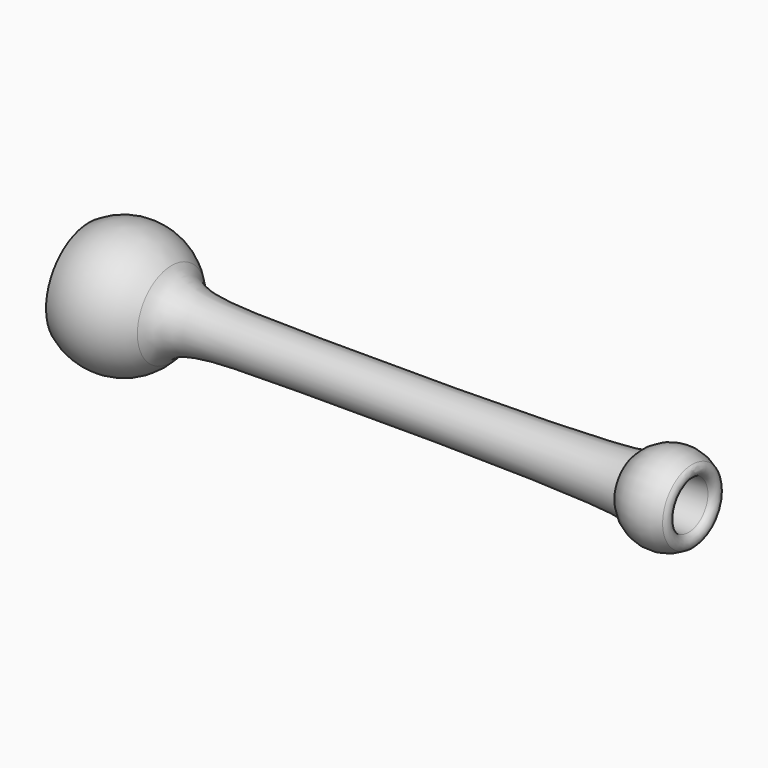
from build123d import *

# Parameters (mm, degrees)
F2_R = 2


# Not quite as in the source:
# - a fillet or chamfer that OpenCascade refuses, or shapes differently, is made with other operations: its cross-section is extruded or revolved along the edge and cut away or added


with BuildPart() as f1:
    # F0 (on Front) → F1 (revolve)
    with BuildSketch(Plane.XZ):
        with BuildLine():
            ThreePointArc((-7.0685046336, 10.3095219212), (4.6853520259, 11.5886788028), (12.2474487139, 2.5))
            Line((12.2474487139, 2.5), (74.2474487139, 2.5))
            Line((74.2474487139, 2.5), (167.5172053195, 7.1876591082))
            ThreePointArc((167.5172053195, 7.1876591082), (158.2467343848, 12.5880657376), (148.3624236969, 8.4159649071))
            add(Edge.make_bspline(
                [(13.7809895682, 12.3177978136), (16.9604661176, 7.0744322303), (43.0476593441, 6.206811463), (139.6269473455, 6.3661232123), (148.3624236969, 8.4159649071)],
                knots=[0, 0, 0, 0, 0.3522433177, 1, 1, 1, 1], degree=3))
            ThreePointArc((13.7809895682, 12.3177978136), (2.4835532955, 18.3159979112), (-10.003236638, 15.5428141988))
            Line((-10.003236638, 15.5428141988), (-7.0685046336, 10.3095219212))
        make_face()
    revolve(axis=Axis((35, 0, 0), (1, 0, 0)))

    # F2
    f2_edges = [f1.edges().sort_by_distance(p)[0] for p in [
        (167.517205, 0, -7.187659),
        (-7.068505, 0, -10.309522),
        (12.247449, 0, -2.5),
    ]]
    fillet(f2_edges, radius=F2_R)

    # F3: fillet of radius 5 on 1 edges, made by hand

    # F3_s1 → F3_t2 (revolve, cut)
    with BuildSketch(Plane.XZ):
        with BuildLine():
            ThreePointArc((74.3728590619, 2.5063030181), (74.2474091346, 2.5015760029), (74.1218800737, 2.5))
            Line((74.1218800737, 2.5), (74.1218800737, 2.4))
            Line((74.1218800737, 2.4), (74.2499600867, 2.4))
            Line((74.2499600867, 2.4), (74.3778786416, 2.4064290784))
            Line((74.3778786416, 2.4064290784), (74.3728590619, 2.5063030181))
        make_face()
    revolve(axis=Axis((74.2474487139, 0, 0), (1, 0, 0)), mode=Mode.SUBTRACT)


solid = f1.part
